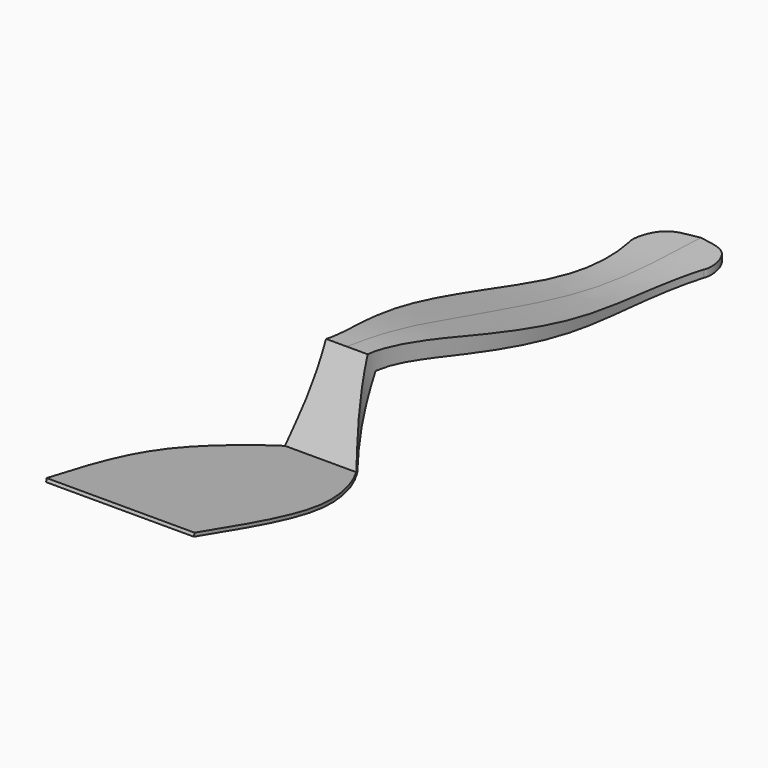
from build123d import *

# Parameters (mm, degrees)
F1_DEPTH = 38.1
F2_W     = 178.1070828438
F2_H     = 414.0989854932
F3_DEPTH = 127


with BuildPart() as f1:
    # F0 (on Right) → F1 (new body, symmetric)
    with BuildSketch(Plane.YZ):
        with BuildLine():
            Line((-121.3063743984, 29.5135372388), (0, 0))
            Line((0, 0), (17.0325431973, 33.8691547513))
            add(Edge.make_bspline(
                [(17.0325431973, 33.8691547513), (25.4235755772, 33.2600981829), (46.9552110301, 29.8717841708), (154.0652576392, 0.5139667568), (198.7675151622, 0.4740691057), (220.6287533045, 0)],
                knots=[0, 0, 0, 0, 0.2237471117, 0.6549288239, 1, 1, 1, 1], degree=3))
            Line((220.6287533045, 0), (220.6287533045, 3.175))
            add(Edge.make_bspline(
                [(220.6287533045, 3.175), (213.7123324331, 3.3744119762), (196.3911320985, 3.9950180389), (147.050553471, 6.466459078), (49.7986920821, 37.8071281556), (22.4555648502, 41.3649031024), (12.2366268188, 42.7516512573)],
                knots=[0, 0, 0, 0, 0.1680141363, 0.421284516, 0.7833399124, 1, 1, 1, 1], degree=3))
            Line((12.2366268188, 42.7516512573), (-3.1861555763, 2.4089931976))
            Line((-3.1861555763, 2.4089931976), (-120.9310872556, 31.0560403378))
            Line((-120.9310872556, 31.0560403378), (-121.3063743984, 29.5135372388))
        make_face()
    extrude(amount=F1_DEPTH, both=True)

    # F2 (on Top) → F3 (cut)
    with BuildSketch(Plane.XY):
        with Locations((-4.5116916299, 43.5459576547)):
            Rectangle(F2_W, F2_H)
        with BuildLine():
            add(Edge.make_bspline(
                [(0, 220.659121871), (-4.9783730098, 219.5793351695), (-16.2285821631, 219.3736032497), (-18.9172811806, 203.3627927303), (-17.5526812673, 200.5418539047)],
                knots=[0, 0, 0, 0, 0.4970280638, 1, 1, 1, 1], degree=3))
            add(Edge.make_bspline(
                [(0, 220.659121871), (4.9783730098, 219.5793351695), (16.2285821631, 219.3736032497), (18.9172811806, 203.3627927303), (17.5526812673, 200.5418539047)],
                knots=[0, 0, 0, 0, 0.4970280638, 1, 1, 1, 1], degree=3))
            add(Edge.make_bspline(
                [(17.5526812673, 200.5418539047), (11.287689209, 174.1361021996), (21.0254121163, 127.5438873027), (20.9275861823, 66.4533676137), (5.1875520429, 11.5580057298), (18.6788079834, -4.1864679667), (42.5575784076, -49.7433913949), (37.3010611033, -95.3904856481), (34.8016284406, -121.3063743984)],
                knots=[0, 0, 0, 0, 0.1974878355, 0.3808250808, 0.5465061702, 0.6447780397, 0.8026257157, 1, 1, 1, 1], degree=3))
            Line((34.8016284406, -121.3063743984), (0, -121.3063743984))
            Line((0, -121.3063743984), (-34.8016284406, -121.3063743984))
            add(Edge.make_bspline(
                [(-17.5526812673, 200.5418539047), (-11.287689209, 174.1361021996), (-21.0254121163, 127.5438873027), (-20.9275861823, 66.4533676137), (-5.1875520429, 11.5580057298), (-18.6788079834, -4.1864679667), (-42.5575784076, -49.7433913949), (-37.3010611033, -95.3904856481), (-34.8016284406, -121.3063743984)],
                knots=[0, 0, 0, 0, 0.1974878355, 0.3808250808, 0.5465061702, 0.6447780397, 0.8026257157, 1, 1, 1, 1], degree=3))
        make_face(mode=Mode.SUBTRACT)
    extrude(amount=F3_DEPTH, mode=Mode.SUBTRACT)


solid = f1.part
